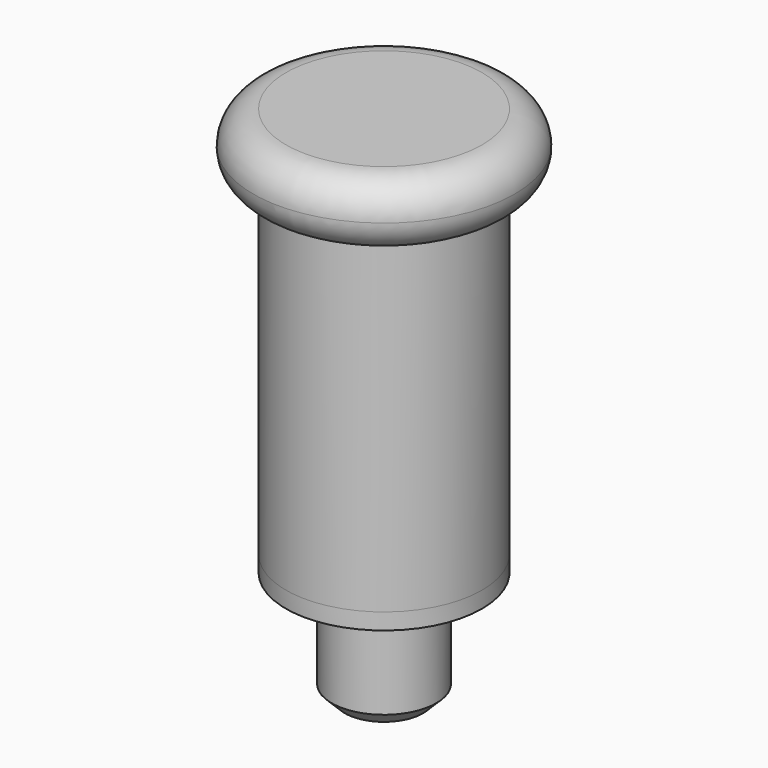
from build123d import *

# Parameters (mm, degrees)
F0_R     = 2
F1_DEPTH = 6
F2_R     = 2
F2_R_2   = 1.5
F2_R_3   = 1.375
F2_R_4   = 0.8
F3_DEPTH = 5
F4_R     = 0.49999
F5_DEPTH = 0.25
F2_R_5   = 0.6
F6_DEPTH = 2
F7_DEPTH = 5.75


# Not quite as in the source:
# - a fillet or chamfer that OpenCascade refuses, or shapes differently, is made with other operations: its cross-section is extruded or revolved along the edge and cut away or added
# - a fillet or chamfer is up to 0.001 mm smaller than in the source, because OpenCascade refuses the exact size


with BuildPart() as f1:
    # F0 (on Top) → F1 (new body)
    with BuildSketch(Plane.XY):
        Circle(F0_R)
    extrude(amount=-F1_DEPTH)

    # F2 (on face) → F3 (cut)
    with BuildSketch(Plane(origin=(0, 0, -6), x_dir=(1, 0, 0), z_dir=(0, 0, -1))):
        Circle(F2_R)
        Circle(F2_R_2, mode=Mode.SUBTRACT)
        Circle(F2_R_3)
        Circle(F2_R_4, mode=Mode.SUBTRACT)
    extrude(amount=-F3_DEPTH, mode=Mode.SUBTRACT)

    # F4 (radius 0.5 in the source; OpenCascade refuses exactly that, so slightly less here)
    f4_edges = [f1.edges().sort_by_distance(p)[0] for p in [
        (-2, 0, 0),
        (-2, 0, -1),
    ]]
    fillet(f4_edges, radius=F4_R)

    # F2 (on face) → F7 (cut)
    with BuildSketch(Plane(origin=(0, 0, -6), x_dir=(1, 0, 0), z_dir=(0, 0, -1))):
        Circle(F2_R_3)
        Circle(F2_R_4, mode=Mode.SUBTRACT)
        Circle(F2_R_4)
        Circle(F2_R_5, mode=Mode.SUBTRACT)
        Circle(F2_R_5)
    extrude(amount=-F7_DEPTH, mode=Mode.SUBTRACT)


with BuildPart() as f5:
    # F2 (on face) → F5 (new body)
    with BuildSketch(Plane(origin=(0, 0, -6), x_dir=(1, 0, 0), z_dir=(0, 0, -1))):
        Circle(F2_R_2)
        Circle(F2_R_3, mode=Mode.SUBTRACT)
        Circle(F2_R_3)
        Circle(F2_R_4, mode=Mode.SUBTRACT)
    extrude(amount=F5_DEPTH)


with BuildPart() as f6:
    # F2 (on face) → F6 (new body)
    with BuildSketch(Plane(origin=(0, 0, -6), x_dir=(1, 0, 0), z_dir=(0, 0, -1))):
        Circle(F2_R_4)
        Circle(F2_R_5, mode=Mode.SUBTRACT)
    extrude(amount=F6_DEPTH)

    # F8: chamfer of 0.25 on 1 edges, made by hand

    # F8_s1 → F8_t2 (revolve, cut)
    with BuildSketch(Plane.XZ):
        Polygon((0.8, -7.75), (0.55, -8), (0.8, -8), align=None)
    revolve(axis=Axis((0, 0, -8), (0, 0, -1)), mode=Mode.SUBTRACT)


solid = Compound([f1.part, f5.part, f6.part])
